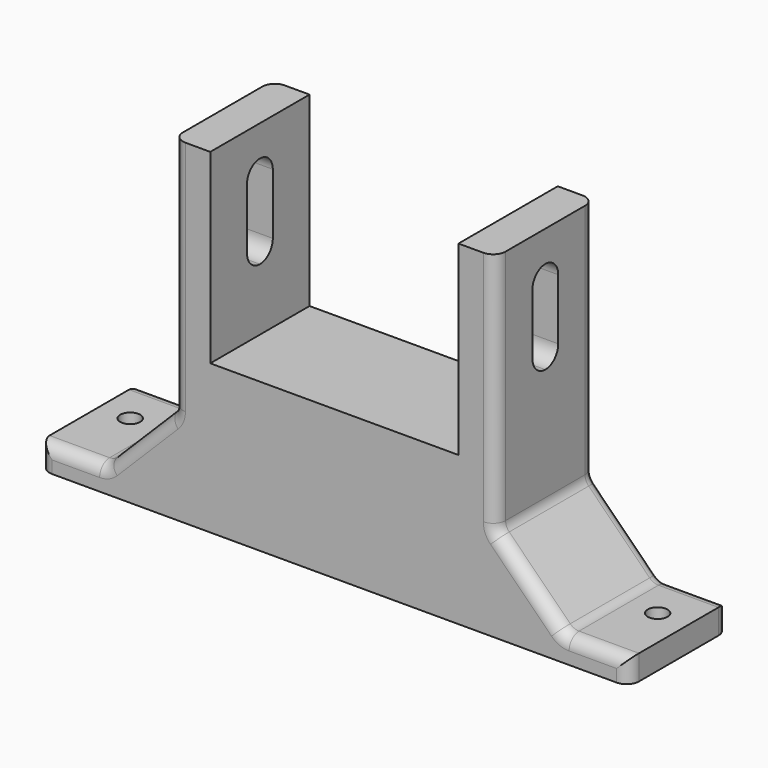
from build123d import *

# Parameters (mm, degrees)
F0_W     = 95
F0_H     = 20
F0_R     = 1.6
F1_DEPTH = 4
F3_DEPTH = 20
F4_SIZE  = 11
F6_DEPTH = 52
F7_F1_R  = 2
F7_F2_R  = 2


with BuildPart() as f1:
    # F0 (on Top) → F1 (new body)
    with BuildSketch(Plane.XY):
        with Locations((0, -2)):
            Rectangle(F0_W, F0_H)
        with Locations((-42.5, 0)):
            Circle(F0_R, mode=Mode.SUBTRACT)
        with Locations((42.5, 0)):
            Circle(F0_R, mode=Mode.SUBTRACT)
    extrude(amount=F1_DEPTH)

    # F2 (on face) → F3 (join, through all)
    with BuildSketch(Plane(origin=(0, 8, 0), x_dir=(-1, 0, 0), z_dir=(0, 1, 0))):
        Polygon((-26, 54), (-26, 4), (26, 4), (26, 54), (20, 54), (20, 24), (-20, 24), (-20, 54), align=None)
    extrude(amount=-F3_DEPTH)

    # F4
    f4_edges = [f1.edges().sort_by_distance(p)[0] for p in [
        (26, -2, 4),
        (-26, -2, 4),
    ]]
    chamfer(f4_edges, length=F4_SIZE)

    # F5 (on face) → F6 (cut, through all)
    with BuildSketch(Plane(origin=(-26, 0, 0), x_dir=(0, -1, 0), z_dir=(-1, 0, 0))):
        with BuildLine():
            ThreePointArc((2, 49), (0.1615223689, 48.2384776311), (-0.6, 46.4))
            Line((-0.6, 46.4), (-0.6, 36.6))
            ThreePointArc((-0.6, 36.6), (0.1615223689, 34.7615223689), (2, 34))
            ThreePointArc((2, 34), (3.8384776311, 34.7615223689), (4.6, 36.6))
            Line((4.6, 36.6), (4.6, 46.4))
            ThreePointArc((4.6, 46.4), (3.8384776311, 48.2384776311), (2, 49))
        make_face()
    extrude(amount=-F6_DEPTH, mode=Mode.SUBTRACT)

    # F7: fillet of radius 2 on 12 edges, made by hand

    # F7_f1
    f7_f1_edges = [f1.edges().sort_by_distance(p)[0] for p in [
        (37, -2, 4),
        (26, -2, 15),
        (-37, -2, 4),
        (-26, -2, 15),
    ]]
    fillet(f7_f1_edges, radius=F7_F1_R)

    # F7_f2
    f7_f2_edges = [f1.edges().sort_by_distance(p)[0] for p in [
        (31.5, 8, 9.5),
        (31.5, -12, 9.5),
        (-31.5, 8, 9.5),
        (-31.5, -12, 9.5),
        (-47.5, -12, 2),
        (-47.5, 8, 2),
        (47.5, -12, 2),
        (47.5, 8, 2),
        (-37.06306026, -12, 4.152240935),
        (-26.152240935, -12, 15.06306026),
        (-37.06306026, 8, 4.152240935),
        (-26.152240935, 8, 15.06306026),
        (37.06306026, -12, 4.152240935),
        (26.152240935, -12, 15.06306026),
        (37.06306026, 8, 4.152240935),
        (26.152240935, 8, 15.06306026),
    ]]
    fillet(f7_f2_edges, radius=F7_F2_R)


solid = f1.part
